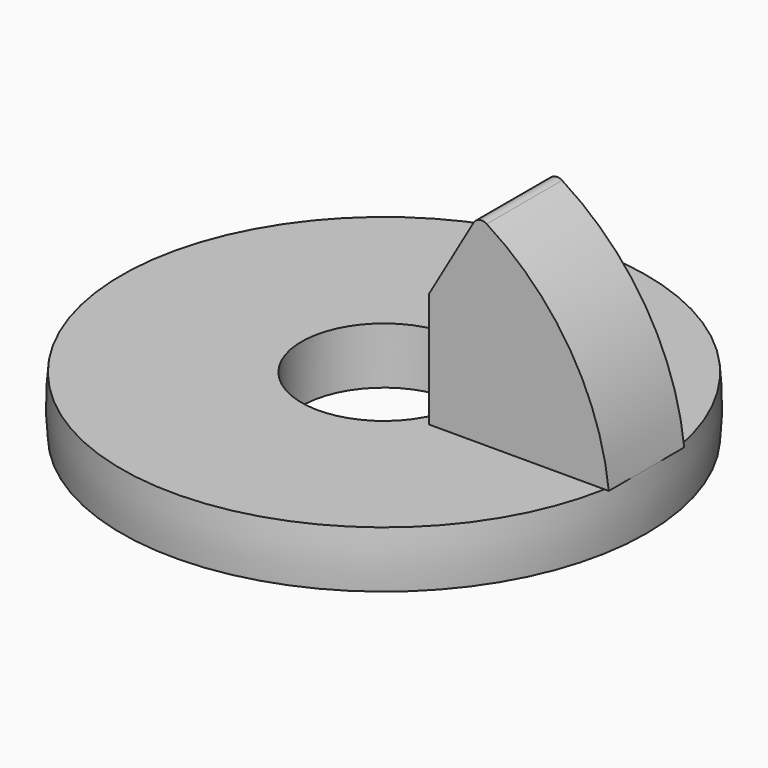
from build123d import *

# Parameters (mm, degrees)
F2_DEPTH = 63.5


# Not quite as in the source:
# - a feature names something its author has since deleted; it is built from what else it names


with BuildPart() as f1:
    # F0 (on Front) → F1 (revolve)
    with BuildSketch(Plane.XZ):
        with BuildLine():
            Line((353.5530370397, 342.9), (111.125, 342.9))
            Line((111.125, 342.9), (111.125, 266.7))
            Line((111.125, 266.7), (353.5530370397, 266.7))
            ThreePointArc((353.5530370397, 266.7), (355.6, 304.8), (353.5530370397, 342.9))
        make_face()
    revolve(axis=Axis((0, 0, 509.3539357185), (0, 0, 1)))

    # F0 (on Front) → F2 (join, symmetric)
    with BuildSketch(Plane.XZ):
        with BuildLine():
            Line((111.125, 497.2741459911), (111.125, 342.9))
            Line((111.125, 342.9), (353.5530370397, 342.9))
            ThreePointArc((353.5530370397, 342.9), (301.5197040525, 493.3132039623), (189.0838855952, 605.9621560027))
            ThreePointArc((189.0838855952, 605.9621560027), (179.2716620853, 607.5323992178), (171.332367053, 601.5563647169))
            Line((171.332367053, 601.5563647169), (111.125, 497.2741459911))
        make_face()
    extrude(amount=F2_DEPTH, both=True)


solid = f1.part
